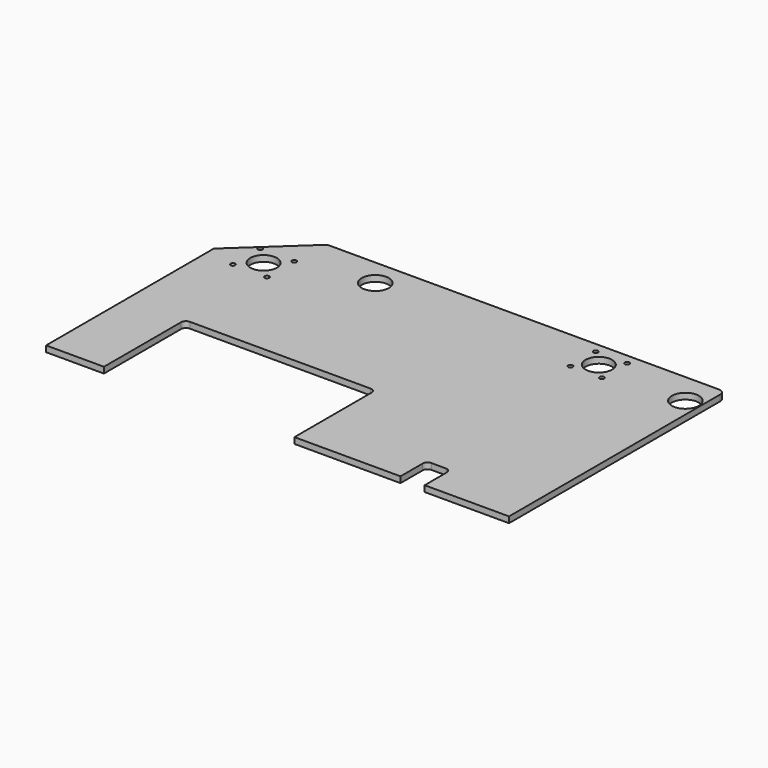
from build123d import *

# Parameters (mm, degrees)
F0_R     = 2.413
F0_R_2   = 13.97
F0_R_3   = 14.2875
F1_DEPTH = 6.35
F2_R     = 5.08


# Not quite as in the source:
# - a length typed as a fraction of an inch, garbled in the dataset ("3 / 203.2 mm" for 3/8 in), is restored


with BuildPart() as f1:
    # F0 (on Top) → F1 (new body)
    with BuildSketch(Plane.XY):
        with BuildLine():
            Line((441.7738245296, 37.0731139821), (29.1392452401, 37.0731139821))
            Line((29.1392452401, 37.0731139821), (-39.5561754704, -26.5958569453))
            Line((-39.5561754704, -26.5958569453), (-39.5561754704, -247.4068860179))
            Line((-39.5561754704, -247.4068860179), (21.4038245296, -247.4068860179))
            Line((21.4038245296, -247.4068860179), (21.4038245296, -140.7268860179))
            Line((21.4038245296, -140.7268860179), (222.0638245296, -140.7268860179))
            Line((222.0638245296, -140.7268860179), (222.0638245296, -247.4068860179))
            Line((222.0638245296, -247.4068860179), (333.8238245296, -247.4068860179))
            Line((333.8238245296, -247.4068860179), (333.8238245296, -213.1168860179))
            Line((333.8238245296, -213.1168860179), (359.2238245296, -213.1168860179))
            Line((359.2238245296, -213.1168860179), (359.2238245296, -247.4068860179))
            Line((359.2238245296, -247.4068860179), (448.1238245296, -247.4068860179))
            Line((448.1238245296, -247.4068860179), (448.1238245296, 30.7231139821))
            ThreePointArc((448.1238245296, 30.7231139821), (446.2639525902, 35.2132420426), (441.7738245296, 37.0731139821))
        make_face()
        with Locations((-9.6586965698, -38.8212736462)):
            Circle(F0_R, mode=Mode.SUBTRACT)
        with Locations((26.2623279145, -38.8212736462)):
            Circle(F0_R, mode=Mode.SUBTRACT)
        with Locations((8.3018156723, -20.860761404)):
            Circle(F0_R_2, mode=Mode.SUBTRACT)
        with Locations((-9.6586965698, -2.9002491619)):
            Circle(F0_R, mode=Mode.SUBTRACT)
        with Locations((26.2623279145, -2.9002491619)):
            Circle(F0_R, mode=Mode.SUBTRACT)
        with Locations((102.5335357666, 8.5151046671)):
            Circle(F0_R_3, mode=Mode.SUBTRACT)
        with Locations((320.4351010724, -6.8675098969)):
            Circle(F0_R, mode=Mode.SUBTRACT)
        with Locations((320.4351010724, 26.3149594916)):
            Circle(F0_R, mode=Mode.SUBTRACT)
        with Locations((353.6175704608, -6.8675098969)):
            Circle(F0_R, mode=Mode.SUBTRACT)
        with Locations((337.0263357666, 9.7237247974)):
            Circle(F0_R_2, mode=Mode.SUBTRACT)
        with Locations((353.6175704608, 26.3149594916)):
            Circle(F0_R, mode=Mode.SUBTRACT)
        with Locations((432.7335357666, 4.0531139821)):
            Circle(F0_R_3, mode=Mode.SUBTRACT)
    extrude(amount=F1_DEPTH)

    # F2
    f2_edges = [f1.edges().sort_by_distance(p)[0] for p in [
        (21.403825, -140.726886, 3.175),
        (222.063825, -140.726886, 3.175),
        (333.823825, -213.116886, 3.175),
        (359.223825, -213.116886, 3.175),
    ]]
    fillet(f2_edges, radius=F2_R)


solid = f1.part
